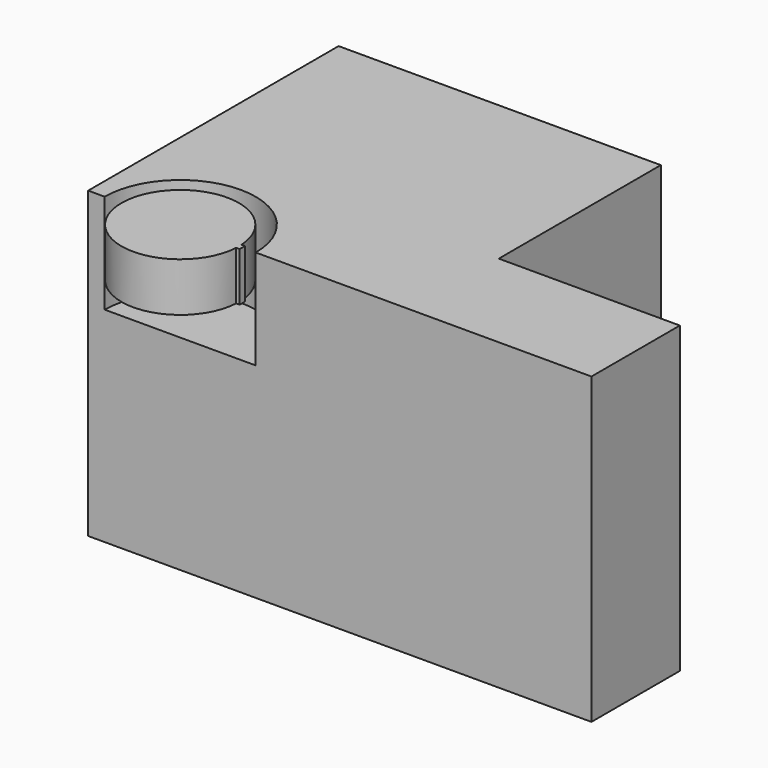
from build123d import *

# Parameters (mm, degrees)
F1_DEPTH    = 25.4
F3_DEPTH    = 8.3058
F4_DEPTH    = 4.0894
F5_W        = 0.9305812418
F5_H        = 0.5637853174
F6_DEPTH    = 4.0894
F7_T        = 2.54
F7_T3_DEPTH = 30.48
F7_T6_ANGLE = 180.000000001


# Not quite as in the source:
# - a shell that OpenCascade refuses in one call is made with other operations: the cavity is built on its own and cut out


with BuildPart() as f1:
    # F0 (on Top) → F1 (new body)
    with BuildSketch(Plane.XY):
        Polygon((-32.2983600199, 26.1462889612), (-32.2983600199, 0), (9.7407754511, 0), (9.7407754511, 9.2281019315), (-5.3830603138, 9.2281019315), (-5.3830603138, 26.1462889612), align=None)
    extrude(amount=F1_DEPTH)

    # F2 (on face) → F3 (cut)
    with BuildSketch(Plane.XY.offset(25.4)):
        with BuildLine():
            Line((-29.5126315491, 0), (-19.7067979438, 0))
            ThreePointArc((-19.7067979438, 0), (-24.6097147465, 4.9029168026), (-29.5126315491, 0))
        make_face()
        with BuildLine():
            Line((-19.7067979438, 0), (-18.3031327531, 0))
            ThreePointArc((-18.3031327531, 0), (-24.6097147465, 6.3065819933), (-30.9162967398, 0))
            Line((-30.9162967398, 0), (-29.5126315491, 0))
            ThreePointArc((-29.5126315491, 0), (-24.6097147465, 4.9029168026), (-19.7067979438, 0))
        make_face()
    extrude(amount=-F3_DEPTH, mode=Mode.SUBTRACT)

    # F7: shell of thickness 2.54, made by hand


with BuildPart() as f4:
    # F2 (on face) → F4 (new body)
    with BuildSketch(Plane.XY.offset(25.4)):
        with BuildLine():
            Line((-29.5126315491, 0), (-19.7067979438, 0))
            ThreePointArc((-19.7067979438, 0), (-24.6097147465, 4.9029168026), (-29.5126315491, 0))
        make_face()
        with BuildLine():
            ThreePointArc((-29.5126315491, 0), (-24.6097147465, -4.9029168026), (-19.7067979438, 0))
            Line((-19.7067979438, 0), (-29.5126315491, 0))
        make_face()
    extrude(amount=-F4_DEPTH)

    # F5 (on face) → F6 (join, through all)
    with BuildSketch(Plane.XY.offset(25.4)):
        with Locations((-19.8902748525, 0)):
            Rectangle(F5_W, F5_H)
    extrude(amount=-F6_DEPTH)


with BuildPart() as f7_core1:
    # F7_t2: copy of F1
    add(f1.part)

    # the walls: a layer under each face that stays
    f7_faces = [f7_core1.faces().sort_by_distance(p)[0] for p in [
        (-32.2983600199, 13.0731444806, 12.7),
        (-18.8407101668, 26.1462889612, 12.7),
        (-11.2787922844, 0, 12.7),
        (-11.2787922844, 13.0731444806, 25.4),
        (-5.3830603138, 17.6871954463, 12.7),
        (9.7407754511, 4.6140509658, 12.7),
        (-24.6097147465, 6.3065819933, 21.2471),
        (-24.6097147465, 3.1532909967, 17.0942),
        (2.1788575687, 9.2281019315, 12.7),
    ]]
    thicken(f7_faces, amount=-F7_T, mode=Mode.SUBTRACT)

    # F7_s4 → F7_t3 (cut)
    with BuildSketch(Plane.XY.offset(-2.54)):
        Polygon((-5.3576603138, 9.2535019315), (-7.9230603138, 9.2281019315), (-7.9230603138, 6.6881019315), (-5.3830603138, 6.6881019315), align=None)
    extrude(amount=F7_T3_DEPTH, mode=Mode.SUBTRACT)

    # F7_s5 → F7_t6 (revolve, cut)
    with BuildSketch(Plane.XZ):
        Polygon((-18.3285327531, 17.1196), (-15.7631327531, 17.0942), (-15.7631327531, 14.5542), (-18.3031327531, 14.5542), align=None)
    revolve(axis=Axis((-24.6097147465, 0, 17.0942), (0, 0, 1)), revolution_arc=F7_T6_ANGLE, mode=Mode.SUBTRACT)


with BuildPart() as f1_1:
    add(f1.part)

    # what is left inside the walls is the cavity
    f7_cavity = [f7_core1.part.solids().sort_by_distance(p)[0] for p in [
        (-11.278792, 2.5654, 15.24),
    ]]
    add(f7_cavity, mode=Mode.SUBTRACT)


solid = Compound([f4.part, f1_1.part])
